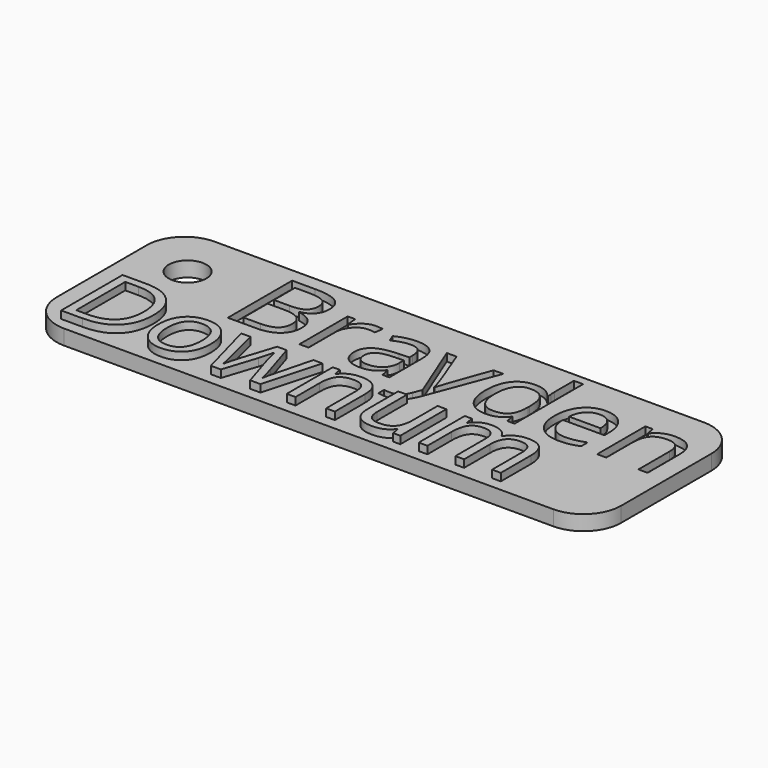
from build123d import *

# Parameters (mm, degrees)
F1_DEPTH     = 2
F3_D         = 5
F4_TEXT_SIZE = 14.9697388729
F5_DEPTH     = 1
F6_TEXT_SIZE = 14.2834364346
F7_DEPTH     = 1


# Not quite as in the source:
# - Text() gives the source's letters only with a copy of the font that has no kerning and outlines rounded to 1/6400 em; it was checked with that copy


with BuildPart() as f1:
    # F0 (on Top) → F1 (new body)
    with BuildSketch(Plane.XY):
        with BuildLine():
            ThreePointArc((37.5, 7.5), (36.0355339059, 11.0355339059), (32.5, 12.5))
            Line((32.5, 12.5), (-32.5, 12.5))
            ThreePointArc((-32.5, 12.5), (-36.0355339059, 11.0355339059), (-37.5, 7.5))
            Line((-37.5, 7.5), (-37.5, -7.5))
            ThreePointArc((-37.5, -7.5), (-36.0355339059, -11.0355339059), (-32.5, -12.5))
            Line((-32.5, -12.5), (32.5, -12.5))
            ThreePointArc((32.5, -12.5), (36.0355339059, -11.0355339059), (37.5, -7.5))
            Line((37.5, -7.5), (37.5, 7.5))
        make_face()
    extrude(amount=F1_DEPTH)

    # F3 (through all)
    with Locations(Plane.XY.offset(2)):
        with Locations((-30.5, 5.5)):
            Hole(F3_D / 2)

    # F4 (on face) → F5 (cut)
    with BuildSketch(Plane.XY.offset(2)):
        with Locations((-22.2203861922, 0)):
            Text('Brayden', F4_TEXT_SIZE, font='Open Sans', text_align=(TextAlign.LEFT, TextAlign.BOTTOM))
    extrude(amount=-F5_DEPTH, mode=Mode.SUBTRACT)

    # F6 (on face) → F7 (join)
    with BuildSketch(Plane.XY.offset(2)):
        with Locations((-35.4803688824, -11.01815328)):
            Text('Downum', F6_TEXT_SIZE, font='Open Sans', text_align=(TextAlign.LEFT, TextAlign.BOTTOM))
    extrude(amount=F7_DEPTH)


solid = f1.part
